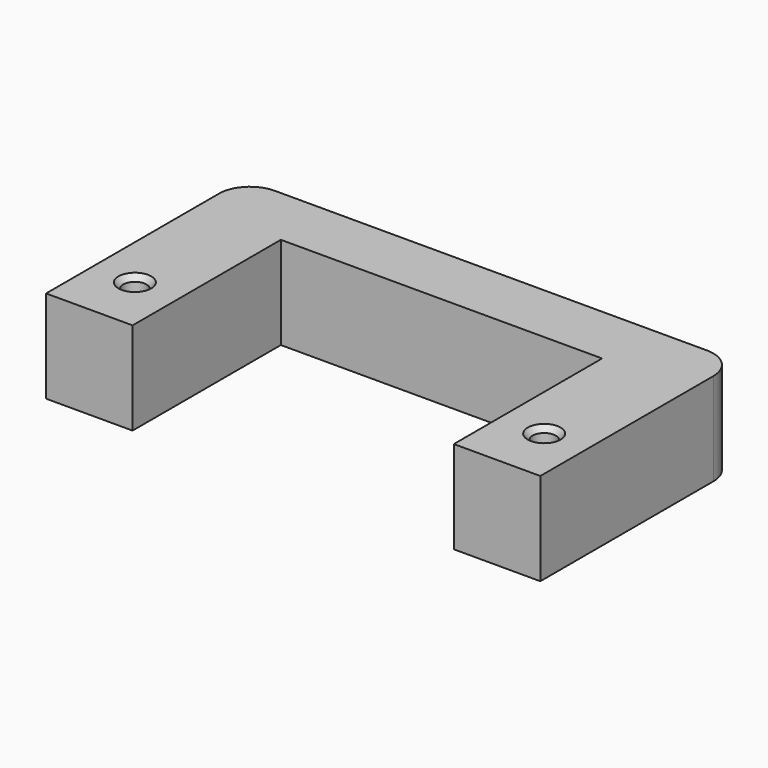
from build123d import *

# Parameters (mm, degrees)
F0_W           = 35.56
F0_H           = 76.2
F1_DEPTH       = 38.1
F3_D           = 9.525
F3_CSINK_D     = 13.4874
F3_CSINK_ANGLE = 82


# Not quite as in the source:
# - a length typed as a fraction of an inch, garbled in the dataset ("3 / 203.2 mm" for 3/8 in), is restored


with BuildPart() as f1:
    # F0 (on Top) → F1 (new body)
    with BuildSketch(Plane.XY):
        with BuildLine():
            Line((97.53417238, 58.7352159441), (-80.26582762, 58.7352159441))
            ThreePointArc((-80.26582762, 58.7352159441), (-89.2460837411, 55.0154720651), (-92.96582762, 46.0352159441))
            Line((-92.96582762, 46.0352159441), (-92.96582762, 33.3352159441))
            Line((-92.96582762, 33.3352159441), (-57.40582762, 33.3352159441))
            Line((-57.40582762, 33.3352159441), (74.67417238, 33.3352159441))
            Line((74.67417238, 33.3352159441), (110.23417238, 33.3352159441))
            Line((110.23417238, 33.3352159441), (110.23417238, 46.0352159441))
            ThreePointArc((110.23417238, 46.0352159441), (106.514428501, 55.0154720651), (97.53417238, 58.7352159441))
        make_face()
        with Locations((-75.18582762, -4.7647840559)):
            Rectangle(F0_W, F0_H)
        with Locations((92.45417238, -4.7647840559)):
            Rectangle(F0_W, F0_H)
    extrude(amount=F1_DEPTH)

    # F3 (through all)
    with Locations(Plane.XY.offset(38.1)):
        with Locations((-75.50332762, -19.0544008167), (92.77167238, -19.0544008167)):
            CounterSinkHole(F3_D / 2, F3_CSINK_D / 2, counter_sink_angle=F3_CSINK_ANGLE)


solid = f1.part
